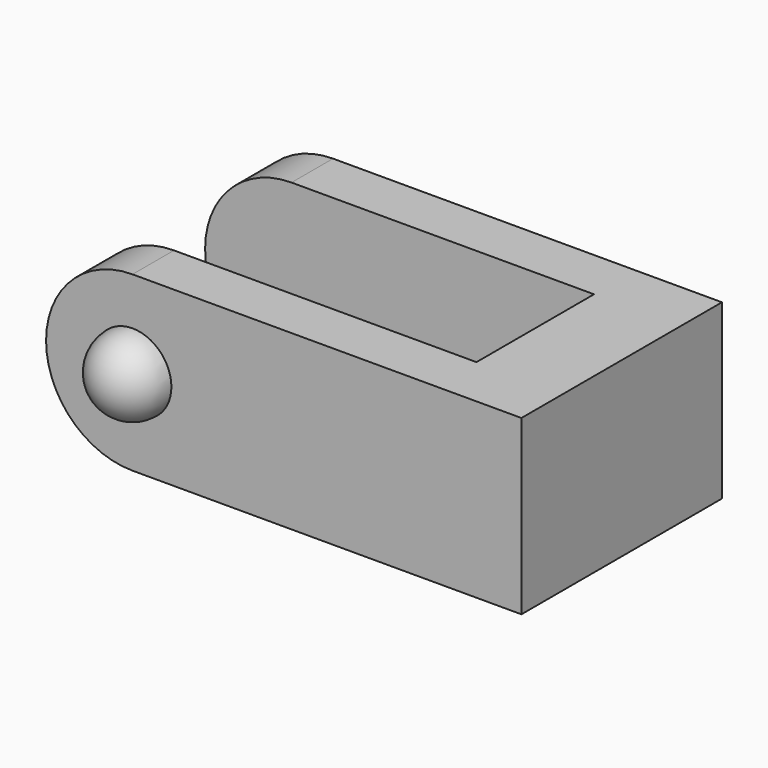
from build123d import *

# Parameters (mm, degrees)
F1_DEPTH = 10
F6_DEPTH = 25


with BuildPart() as f1:
    # F0 (on Top) → F1 (new body)
    with BuildSketch(Plane.XY):
        Polygon((25, 4.25), (25, 0), (30, 0), (30, 7.25), (0, 7.25), (0, 4.25), align=None)
    extrude(amount=F1_DEPTH)

    # F2 (on face) → F3 (revolve)
    with BuildSketch(Plane(origin=(0, 7.25, 0), x_dir=(-1, 0, 0), z_dir=(0, 1, 0))):
        with BuildLine():
            Line((-7.5, 7.25), (-7.5, 2.75))
            ThreePointArc((-7.5, 2.75), (-5.25, 5), (-7.5, 7.25))
        make_face()
    revolve(axis=Axis((7.5, 7.25, 5), (0, 0, -1)))

    # F4: F1 across plane


with BuildPart() as f1_1:
    add(f1.part)
    add(f1.part.mirror(Plane.XZ))

    # F5 (on face) → F6 (cut)
    with BuildSketch(Plane.XZ.offset(7.25)):
        with BuildLine():
            ThreePointArc((7.5, 0), (2.5, 5), (7.5, 10))
            Line((7.5, 10), (0, 10))
            Line((0, 10), (0, 0))
            Line((0, 0), (7.5, 0))
        make_face()
    extrude(amount=-F6_DEPTH, mode=Mode.SUBTRACT)


solid = f1_1.part
